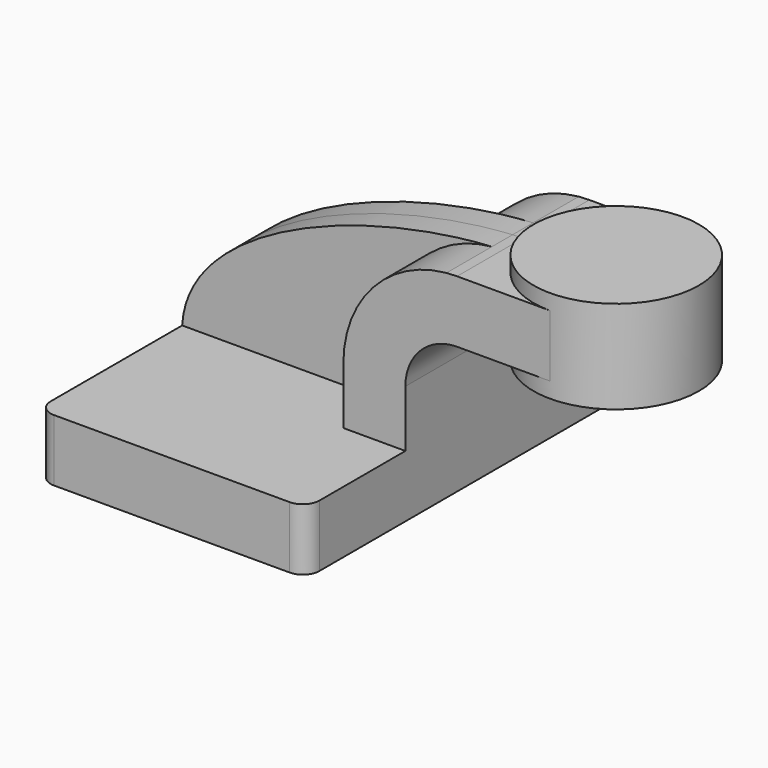
from build123d import *

# Parameters (mm, degrees)
F1_DEPTH     = 63.5
F0_W         = 25.4
F0_H         = 19.05
F2_DEPTH     = 25.4
F3_DEPTH     = 7.9375
F5_R         = 5.08
F6_T         = 5.08
F6_T3_DEPTH  = 29.21
F6_T5_DEPTH  = 27.6225
F6_T7_DEPTH  = 73.66
F6_T9_DEPTH  = 27.6352
F6_T11_DEPTH = 27.6225
F6_T14_ANGLE = 84.6365269518
F6_T16_ANGLE = 180.000000001
F6_T18_ANGLE = 180.000000001
F6_T20_ANGLE = 84.6365269518


# Not quite as in the source:
# - a shell that OpenCascade refuses in one call is made with other operations: the cavity is built on its own and cut out


with BuildPart() as f1:
    # F0 (on Front) → F1 (new body, symmetric)
    with BuildSketch(Plane.XZ):
        Polygon((22.225, 9.525), (-41.275, 9.525), (-41.275, -9.525), (41.275, -9.525), (41.275, 9.525), align=None)
    extrude(amount=F1_DEPTH, both=True)

    # F0 (on Front) → F2 (join, symmetric)
    with BuildSketch(Plane.XZ):
        with BuildLine():
            Line((22.225, 27.0002), (22.225, 9.525))
            Line((22.225, 9.525), (41.275, 9.525))
            Line((41.275, 9.525), (41.275, 27.0002))
            ThreePointArc((41.275, 27.0002), (45.9246798487, 38.2255201513), (57.15, 42.8752))
            Line((57.15, 42.8752), (60.325, 42.8752))
            Line((60.325, 42.8752), (60.325, 61.9252))
            Line((60.325, 61.9252), (57.15, 61.9252))
            add(Edge.make_bspline(
                [(53.8854342407, 61.7722898912), (54.9842067368, 61.8365871986), (56.0728453275, 61.8876096574), (57.15, 61.9252)],
                knots=[108.5245810491, 108.5245810491, 108.5245810491, 108.5245810491, 111.5045361635, 111.5045361635, 111.5045361635, 111.5045361635], degree=3))
            ThreePointArc((53.8854342407, 61.7722898912), (31.3258777096, 50.5133948686), (22.225, 27.0002))
        make_face()
        with Locations((73.025, 52.4002)):
            Rectangle(F0_W, F0_H)
    extrude(amount=F2_DEPTH, both=True)

    # F0 (on Front) → F3 (join, symmetric)
    with BuildSketch(Plane.XZ):
        with BuildLine():
            add(Edge.make_bspline(
                [(-41.275, 9.525), (-39.5856284224, 39.4828766469), (13.870125209, 59.4306981306), (53.8854342407, 61.7722898912)],
                knots=[0, 0, 0, 0, 108.5245810491, 108.5245810491, 108.5245810491, 108.5245810491], degree=3))
            Line((-41.275, 9.525), (22.225, 9.525))
            Line((22.225, 9.525), (22.225, 27.0002))
            ThreePointArc((22.225, 27.0002), (31.3258777096, 50.5133948686), (53.8854342407, 61.7722898912))
        make_face()
    extrude(amount=F3_DEPTH, both=True)

    # F0 (on Front) → F4 (revolve)
    with BuildSketch(Plane.XZ):
        Polygon((85.725, 66.675), (85.725, 61.9252), (85.725, 42.8752), (85.725, 38.1), (111.125, 38.1), (111.125, 66.675), align=None)
    revolve(axis=Axis((85.725, 0, 52.3875), (0, 0, 1)))

    # F5
    f5_edges = [f1.edges().sort_by_distance(p)[0] for p in [
        (41.275, -63.5, 0),
        (-41.275, -63.5, 0),
        (41.275, 63.5, 0),
        (-41.275, 63.5, 0),
    ]]
    fillet(f5_edges, radius=F5_R)

    # F6: shell of thickness 5.08, made by hand


with BuildPart() as f6_core1:
    # F6_t2: copy of F1
    add(f1.part)

    # the walls: a layer under each face that stays
    f6_faces = [f6_core1.faces().sort_by_distance(p)[0] for p in [
        (0, 35.71875, 9.525),
        (41.275, 0, 8.7376),
        (32.8083333333, 25.4, 18.2583666667),
        (0, 63.5, 0),
        (22.225, 16.66875, 18.2626),
        (6.3052171204, 7.9375, 35.6486449456),
        (-41.275, 0, 0),
        (45.9246798487, 0, 38.2255201513),
        (32.8083333333, -25.4, 18.2583666667),
        (0, -35.71875, 9.525),
        (31.3258777096, 16.66875, 50.5133948686),
        (61.9125, 16.9333333333, 42.8752),
        (98.425, 21.9970452561, 42.8625),
        (61.9125, 16.9333333333, 61.9252),
        (55.5258238042, 12.7, 61.8587600574),
        (-8.0670094249, 3.96875, 46.0047517779),
        (-8.0670094249, -3.96875, 46.0047517779),
        (0, -63.5, 0),
        (31.3258777096, -16.66875, 50.5133948686),
        (22.225, -16.66875, 18.2626),
        (55.5258238042, -12.7, 61.8587600574),
        (6.3052171204, -7.9375, 35.6486449456),
        (85.725, 0, 66.675),
    ]]
    thicken(f6_faces, amount=-F6_T, mode=Mode.SUBTRACT)

    # F6_s4 → F6_t3 (cut)
    with BuildSketch(Plane.YZ.offset(17.145)):
        Polygon((25.4508, 9.5758), (25.4, 4.445), (20.32, 4.445), (20.32, 9.525), align=None)
        Polygon((-25.4508, 9.5758), (-20.32, 9.525), (-20.32, 4.445), (-25.4, 4.445), align=None)
    extrude(amount=F6_T3_DEPTH, mode=Mode.SUBTRACT)

    # F6_s6 → F6_t5 (cut)
    with BuildSketch(Plane.XZ.offset(-30.48)):
        Polygon((22.1742, 9.5758), (22.225, 4.445), (27.305, 4.445), (27.305, 9.525), align=None)
    extrude(amount=F6_T5_DEPTH, mode=Mode.SUBTRACT)

    # F6_s8 → F6_t7 (cut)
    with BuildSketch(Plane.YZ.offset(-46.355)):
        Polygon((7.9883, 9.5758), (7.9375, 4.445), (2.8575, 4.445), (2.8575, 9.525), align=None)
        Polygon((-7.9883, 9.5758), (-7.9375, 4.445), (-2.8575, 4.445), (-2.8575, 9.525), align=None)
    extrude(amount=F6_T7_DEPTH, mode=Mode.SUBTRACT)

    # F6_s10 → F6_t9 (cut)
    with BuildSketch(Plane.XY.offset(4.445)):
        Polygon((22.1742, 7.9883), (27.305, 7.9375), (27.305, 2.8575), (22.225, 2.8575), align=None)
        Polygon((22.1742, -7.9883), (27.305, -7.9375), (27.305, -2.8575), (22.225, -2.8575), align=None)
    extrude(amount=F6_T9_DEPTH, mode=Mode.SUBTRACT)

    # F6_s12 → F6_t11 (cut)
    with BuildSketch(Plane.XZ.offset(2.8575)):
        Polygon((22.1742, 9.5758), (22.225, 4.445), (27.305, 4.445), (27.305, 9.525), align=None)
    extrude(amount=F6_T11_DEPTH, mode=Mode.SUBTRACT)

    # F6_s13 → F6_t14 (revolve, cut)
    with BuildSketch(Plane.XY.offset(27.0002)):
        Polygon((22.1742, 7.9883), (22.225, 2.8575), (27.305, 2.8575), (27.305, 7.9375), align=None)
    revolve(axis=Axis((57.15, 7.9375, 27.0002), (0, 1, 0)), revolution_arc=F6_T14_ANGLE, mode=Mode.SUBTRACT)

    # F6_s15 → F6_t16 (revolve, cut)
    with BuildSketch(Plane.YZ.offset(85.725)):
        Polygon((25.4508, 42.8244), (25.4, 47.9552), (20.32, 47.9552), (20.32, 42.8752), align=None)
    revolve(axis=Axis((85.725, 0, 42.8752), (0, 0, 1)), revolution_arc=F6_T16_ANGLE, mode=Mode.SUBTRACT)

    # F6_s17 → F6_t18 (revolve, cut)
    with BuildSketch(Plane.YZ.offset(85.725)):
        Polygon((25.4508, 61.976), (20.32, 61.9252), (20.32, 56.8452), (25.4, 56.8452), align=None)
    revolve(axis=Axis((85.725, 0, 61.9252), (0, 0, 1)), revolution_arc=F6_T18_ANGLE, mode=Mode.SUBTRACT)

    # F6_s19 → F6_t20 (revolve, cut)
    with BuildSketch(Plane.XY.offset(27.0002)):
        Polygon((22.1742, -7.9883), (27.305, -7.9375), (27.305, -2.8575), (22.225, -2.8575), align=None)
    revolve(axis=Axis((57.15, -7.9375, 27.0002), (0, 1, 0)), revolution_arc=F6_T20_ANGLE, mode=Mode.SUBTRACT)


with BuildPart() as f1_1:
    add(f1.part)

    # what is left inside the walls is the cavity
    f6_cavity = [f6_core1.part.solids().sort_by_distance(p)[0] for p in [
        (0, 19.473333, -9.4742),
    ]]
    add(f6_cavity, mode=Mode.SUBTRACT)


solid = f1_1.part
